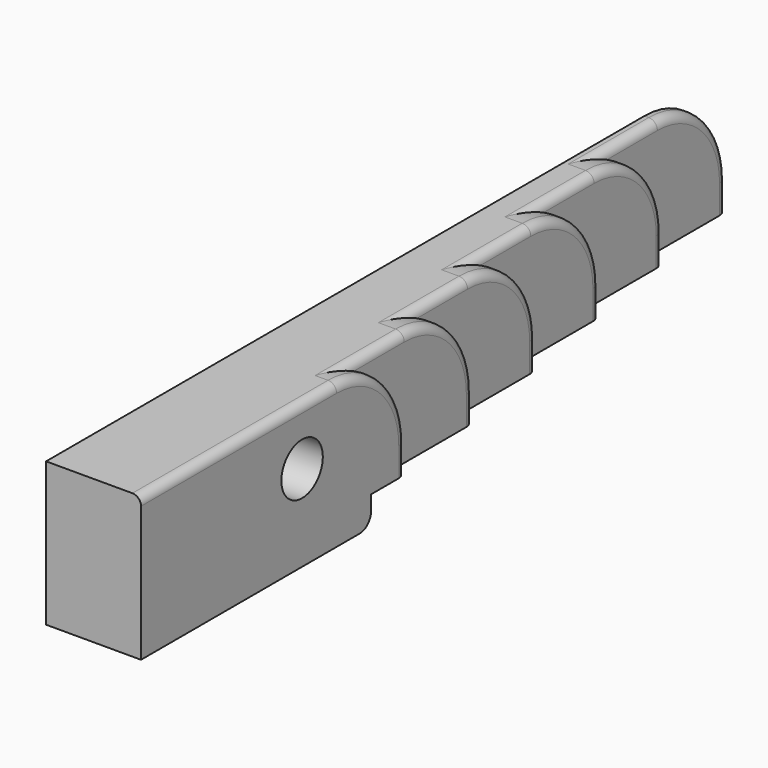
from build123d import *

# Parameters (mm, degrees)
F0_W     = 6.6
F0_H     = 14
F1_DEPTH = 8
F2_DEPTH = 2
F3_R     = 1.8
F4_DEPTH = 6.6
F5_R     = 6
F6_R     = 0.6
F7_DEPTH = 6
F8_R     = 1


with BuildPart() as f1:
    # F0 (on Top) → F1 (new body)
    with BuildSketch(Plane.XY):
        with Locations((0, -22)):
            Rectangle(F0_W, F0_H)
        Polygon((-3.3, -15), (3.3, -15), (3.3, -6), (2.4, -6), (2.4, 1), (1.2, 1), (1.2, 8), (0, 8), (0, 15), (-1.2, 15), (-1.2, 22), (-2.4, 22), (-2.4, 29), (-3.3, 29), align=None)
    extrude(amount=F1_DEPTH)

    # F0 (on Top) → F2 (join)
    with BuildSketch(Plane.XY):
        with Locations((0, -22)):
            Rectangle(F0_W, F0_H)
    extrude(amount=-F2_DEPTH)

    # F3 (on face) → F4 (cut)
    with BuildSketch(Plane.YZ.offset(3.3)):
        with Locations((-15, 4)):
            Circle(F3_R)
    extrude(amount=-F4_DEPTH, mode=Mode.SUBTRACT)

    # F5
    f5_edges = [f1.edges().sort_by_distance(p)[0] for p in [
        (2.85, -6, 8),
        (1.8, 1, 8),
        (0.6, 8, 8),
        (-0.6, 15, 8),
        (-1.8, 22, 8),
        (-2.85, 29, 8),
    ]]
    fillet(f5_edges, radius=F5_R)

    # F6
    f6_edges = [f1.edges().sort_by_distance(p)[0] for p in [
        (-2.4, 27.242641, 6.242641),
        (-2.4, 29, 1),
        (3.3, -20.5, 8),
        (2.4, -9, 8),
        (2.4, -5.5, 8),
        (-2.4, 22.5, 8),
        (1.2, -2, 8),
        (-2.4, 19, 8),
        (1.2, 1.5, 8),
        (-1.2, 15.5, 8),
        (0, 5, 8),
        (-1.2, 12, 8),
        (0, 8.5, 8),
        (-1.2, 22, 1),
        (-1.2, 20.242641, 6.242641),
        (0, 15, 1),
        (0, 13.242641, 6.242641),
        (1.2, 8, 1),
        (1.2, 6.242641, 6.242641),
        (2.4, 1, 1),
        (2.4, -0.757359, 6.242641),
        (3.3, -6, 1),
        (3.3, -7.757359, 6.242641),
    ]]
    fillet(f6_edges, radius=F6_R)

    # F7 (add): a face of the model
    f7_faces = [f1.faces().sort_by_distance(p)[0] for p in [
        (0, -15, -1),
    ]]
    extrude(f7_faces, amount=F7_DEPTH)

    # F8
    f8_edges = [f1.edges().sort_by_distance(p)[0] for p in [
        (0, -9, -2),
    ]]
    fillet(f8_edges, radius=F8_R)


solid = f1.part
